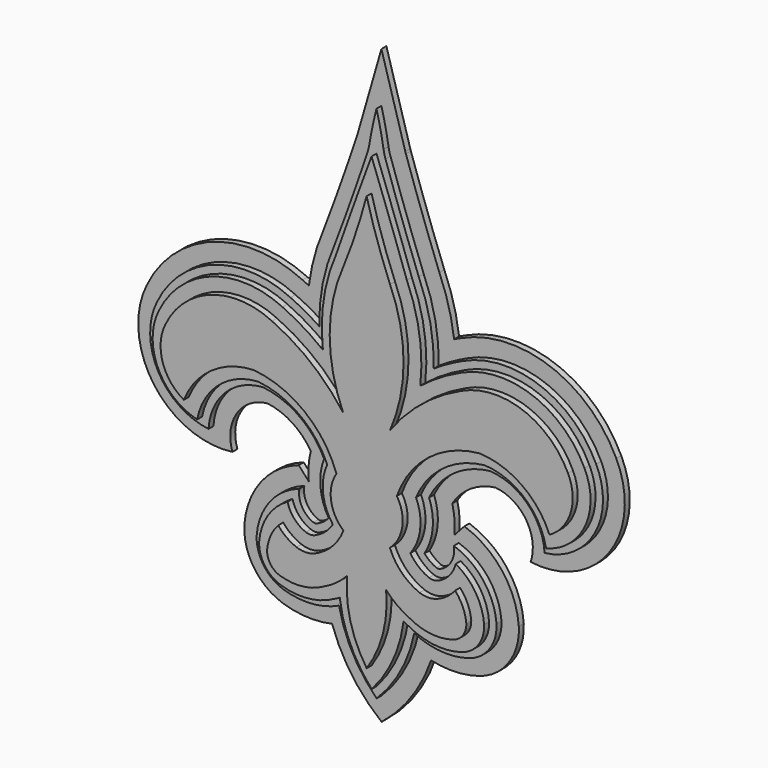
from build123d import *

# Parameters (mm, degrees)
F1_DEPTH    = 25.4
F2_DEPTH    = 19.05
F3_DEPTH    = 12.7
F4_DEPTH    = 6.35
F5_R        = 50.8
F6_T1_DEPTH = 6.35


# Not quite as in the source:
# - a fillet or chamfer that OpenCascade refuses, or shapes differently, is made with other operations: its cross-section is extruded or revolved along the edge and cut away or added


with BuildPart() as f1:
    # F0 (on Front) → F1 (new body)
    with BuildSketch(Plane.XZ):
        with BuildLine():
            ThreePointArc((-107.6217740774, 8.690867573), (-55.6471023956, -11.8476623191), (-22.9876432568, -57.196944952))
            ThreePointArc((-22.9876432568, -57.196944952), (-28.5301171317, -83.0656311724), (-15.8199295402, -106.268197298))
            ThreePointArc((-15.8199295402, -106.268197298), (-27.8174961879, -124.6891161431), (-46.1557023227, -136.8127316236))
            ThreePointArc((-46.1557023227, -136.8127316236), (-55.0099629909, -138.3229508994), (-63.864223659, -136.8127316236))
            ThreePointArc((-63.864223659, -136.8127316236), (-74.1425982594, -131.2503429818), (-82.5992301113, -123.1837123623))
            ThreePointArc((-82.5992301113, -123.1837123623), (-90.4911472712, -135.2405064996), (-94.0484032041, -149.2045521727))
            ThreePointArc((-94.0484032041, -149.2045521727), (-90.7020512597, -160.6634696416), (-81.1531394727, -167.8274869909))
            ThreePointArc((-81.1531394727, -167.8274869909), (-58.036080583, -170.2020518531), (-35.9072424478, -163.1061732759))
            ThreePointArc((-35.9072424478, -163.1061732759), (-23.0493888803, -155.5361787921), (-11.9526460775, -145.5616354935))
            ThreePointArc((-11.9526460775, -145.5616354935), (-8.6762501422, -185.8257002735), (8.0091749091, -222.6160016284))
            ThreePointArc((8.0091749091, -222.6160016284), (24.6729779001, -185.8159017262), (27.9257127936, -145.5499185811))
            ThreePointArc((27.9257127936, -145.5499185811), (39.028315047, -155.51793935), (51.8906147699, -163.0803768332))
            ThreePointArc((51.8906147699, -163.0803768332), (74.0236188538, -170.163250559), (97.1392783805, -167.77510177))
            ThreePointArc((97.1392783805, -167.77510177), (106.6839787089, -160.605474406), (110.0235964424, -149.1445924901))
            ThreePointArc((110.0235964424, -149.1445924901), (106.4581353955, -135.1826395875), (98.5591346332, -123.1304850794))
            ThreePointArc((98.5591346332, -123.1304850794), (90.1072444563, -131.2020836985), (79.8321402713, -136.7705112878))
            ThreePointArc((79.8321402713, -136.7705112878), (70.9787685859, -138.2859333548), (62.1236219925, -136.7809173918))
            ThreePointArc((62.1236219925, -136.7809173918), (43.7782947925, -124.6680801317), (31.7699054842, -106.2542146282))
            ThreePointArc((31.7699054842, -106.2542146282), (44.4664562975, -83.0441835883), (38.9087820968, -57.1787587725))
            ThreePointArc((38.9087820968, -57.1787587725), (71.541586881, -11.8102922073), (123.5041804799, 8.7587761489))
            ThreePointArc((123.5041804799, 8.7587761489), (166.7993623153, -5.6625752644), (195.2107705111, -41.3730783563))
            ThreePointArc((195.2107705111, -41.3730783563), (216.9732861452, -14.2511624984), (214.1399674952, 20.4068482921))
            ThreePointArc((214.1399674952, 20.406848292), (167.4978613851, 62.4099195769), (104.8241776257, 58.9815929048))
            ThreePointArc((104.8241776257, 58.9815929048), (64.5980000023, 34.2064244966), (31.9967480605, 0.0141343178))
            ThreePointArc((31.9967480605, 0.0141343178), (45.7550134481, 65.6656974668), (31.9195995813, 131.3010456682))
            ThreePointArc((31.9195995813, 131.3010456682), (18.7586509593, 166.8011753165), (7.884102283, 203.0670541114))
            ThreePointArc((7.884102283, 203.0670541115), (-2.9691335039, 166.7947913391), (-16.109218821, 131.2869340179))
            ThreePointArc((-16.109218821, 131.2869340178), (-29.9060608303, 65.6434670089), (-16.109218821, 0))
            ThreePointArc((-16.109218821, 0), (-48.7305576375, 34.1731267177), (-88.9712870116, 58.9246526358))
            ThreePointArc((-88.9712870116, 58.9246526358), (-151.6469745465, 62.3161496178), (-198.2643902305, 20.285677164))
            ThreePointArc((-198.2643902306, 20.285677164), (-201.0773422152, -14.3739925929), (-179.2988926172, -41.4831154048))
            ThreePointArc((-179.2988926172, -41.4831154048), (-150.9084739818, -5.7559230095), (-107.6217740774, 8.690867573))
        make_face()
    extrude(amount=F1_DEPTH)


with BuildPart() as f2:
    # F0 (on Front) → F2 (new body)
    with BuildSketch(Plane.XZ):
        with BuildLine():
            ThreePointArc((-29.8756994534, -174.8675902704), (-27.2540366228, -173.5851626194), (-24.6763913381, -172.2164108292))
            ThreePointArc((-24.6763913381, -172.2164108292), (-13.8552320974, -210.6071310198), (8.0154470243, -243.9630642074))
            ThreePointArc((8.0154470244, -243.9630642076), (29.8665213371, -210.5942848556), (40.6651190717, -172.1972124277))
            ThreePointArc((40.6651190717, -172.1972124277), (43.2435682345, -173.5644492733), (45.8659842087, -174.8453361284))
            ThreePointArc((45.8659842087, -174.8453361284), (72.9824435341, -183.3333720605), (101.2373155697, -180.3314848901))
            ThreePointArc((101.2373155697, -180.3314848901), (117.6139086806, -168.0214032355), (123.207807962, -148.3125422056))
            ThreePointArc((123.207807962, -148.3125422056), (114.3375630575, -122.0268333634), (94.1184470923, -103.0319107896))
            ThreePointArc((94.1184470923, -103.0319107896), (87.3104303405, -115.9909745964), (75.3015691391, -124.3619768951))
            ThreePointArc((75.3015691391, -124.3619768951), (71.0179091203, -125.077827485), (66.7285761619, -124.3967929812))
            ThreePointArc((66.7285761619, -124.3967929812), (55.960270597, -117.9342540793), (47.6625489032, -108.5072381948))
            ThreePointArc((47.6625489032, -108.5072381948), (57.7611970568, -83.1911033438), (53.4239364189, -56.2824142549))
            ThreePointArc((53.4239364189, -56.2824142549), (81.5889270302, -20.7682056521), (123.8857690009, -4.4739469049))
            ThreePointArc((123.8857690009, -4.4739469049), (164.7280810138, -20.7728810464), (186.6525395472, -58.8920077772))
            ThreePointArc((186.6525395472, -58.8920077772), (226.6750123427, -25.770970788), (226.0223289435, 26.1749185998))
            ThreePointArc((226.0223289435, 26.1749185998), (171.9221419751, 74.8549107017), (99.249087183, 70.9563252865))
            ThreePointArc((99.249087183, 70.9563252865), (77.767380419, 59.6132449174), (57.8415310441, 45.7175720496))
            ThreePointArc((57.8415310441, 45.7175720496), (56.970930759, 91.9956374625), (44.0833550857, 136.4515445669))
            ThreePointArc((44.0833550857, 136.4515445669), (26.2240315586, 186.4788338094), (7.8743295738, 236.3283427626))
            ThreePointArc((7.8743295738, 236.3283427626), (-10.4460760474, 186.4680595336), (-28.2759988262, 136.4302842083))
            ThreePointArc((-28.275998826, 136.4302842085), (-41.1374485351, 91.9668116204), (-41.9808541711, 45.6882426046))
            ThreePointArc((-41.9808541711, 45.6882426046), (-61.9148656556, 59.572203995), (-83.4032342743, 70.902659055))
            ThreePointArc((-83.4032342743, 70.902659055), (-156.0785674547, 74.7585387426), (-210.1501391332, 26.0467640134))
            ThreePointArc((-210.1501391332, 26.0467640134), (-210.772297323, -25.8994999436), (-170.7303684373, -58.9970127055))
            ThreePointArc((-170.7303684373, -58.9970127055), (-148.8283137299, -20.8650090302), (-107.9955865534, -4.5420774297))
            ThreePointArc((-107.9955865534, -4.5420774297), (-65.6891768482, -20.8114783615), (-37.5033217938, -56.3091301665))
            ThreePointArc((-37.5033217938, -56.3091301665), (-41.8247692607, -83.2203633251), (-31.7112462651, -108.5305595104))
            ThreePointArc((-31.7112462651, -108.5305595104), (-40.0034269046, -117.962449779), (-50.7679330119, -124.4313153721))
            ThreePointArc((-50.7679330119, -124.4313153721), (-55.0568650317, -125.1148703102), (-59.340944968, -124.401537062))
            ThreePointArc((-59.340944968, -124.401537062), (-71.3547231697, -116.0375930066), (-78.170353914, -103.0825320497))
            ThreePointArc((-78.170353914, -103.0825320497), (-98.378304353, -122.0893327552), (-107.2331013872, -148.3802495038))
            ThreePointArc((-107.2331013872, -148.3802495038), (-101.6276215028, -168.0858199734), (-85.2437974144, -180.386276083))
            ThreePointArc((-85.2437974144, -180.386276083), (-56.9871662505, -183.3715592519), (-29.8756994534, -174.8675902704))
        make_face()
        with BuildLine():
            ThreePointArc((-15.8199295402, -106.268197298), (-28.5301171317, -83.0656311724), (-22.9876432568, -57.196944952))
            ThreePointArc((-22.9876432568, -57.196944952), (-55.6471023956, -11.8476623191), (-107.6217740774, 8.690867573))
            ThreePointArc((-107.6217740774, 8.690867573), (-150.9084739818, -5.7559230095), (-179.2988926172, -41.4831154048))
            ThreePointArc((-179.2988926172, -41.4831154048), (-201.0773422152, -14.3739925929), (-198.2643902306, 20.285677164))
            ThreePointArc((-198.2643902305, 20.285677164), (-151.6469745465, 62.3161496178), (-88.9712870116, 58.9246526358))
            ThreePointArc((-88.9712870116, 58.9246526358), (-48.7305576375, 34.1731267177), (-16.109218821, 0))
            ThreePointArc((-16.109218821, 0), (-29.9060608303, 65.6434670089), (-16.109218821, 131.2869340178))
            ThreePointArc((-16.109218821, 131.2869340179), (-2.9691335039, 166.7947913391), (7.884102283, 203.0670541115))
            ThreePointArc((7.884102283, 203.0670541114), (18.7586509593, 166.8011753165), (31.9195995813, 131.3010456682))
            ThreePointArc((31.9195995813, 131.3010456682), (45.7550134481, 65.6656974668), (31.9967480605, 0.0141343178))
            ThreePointArc((31.9967480605, 0.0141343178), (64.5980000023, 34.2064244966), (104.8241776257, 58.9815929048))
            ThreePointArc((104.8241776257, 58.9815929048), (167.4978613851, 62.4099195769), (214.1399674952, 20.406848292))
            ThreePointArc((214.1399674952, 20.4068482921), (216.9732861452, -14.2511624984), (195.2107705111, -41.3730783563))
            ThreePointArc((195.2107705111, -41.3730783563), (166.7993623153, -5.6625752644), (123.5041804799, 8.7587761489))
            ThreePointArc((123.5041804799, 8.7587761489), (71.541586881, -11.8102922073), (38.9087820968, -57.1787587725))
            ThreePointArc((38.9087820968, -57.1787587725), (44.4664562975, -83.0441835883), (31.7699054842, -106.2542146282))
            ThreePointArc((31.7699054842, -106.2542146282), (43.7782947925, -124.6680801317), (62.1236219925, -136.7809173918))
            ThreePointArc((62.1236219925, -136.7809173918), (70.9787685859, -138.2859333548), (79.8321402713, -136.7705112878))
            ThreePointArc((79.8321402713, -136.7705112878), (90.1072444563, -131.2020836985), (98.5591346332, -123.1304850794))
            ThreePointArc((98.5591346332, -123.1304850794), (106.4581353955, -135.1826395875), (110.0235964424, -149.1445924901))
            ThreePointArc((110.0235964424, -149.1445924901), (106.6839787089, -160.605474406), (97.1392783805, -167.77510177))
            ThreePointArc((97.1392783805, -167.77510177), (74.0236188538, -170.163250559), (51.8906147699, -163.0803768332))
            ThreePointArc((51.8906147699, -163.0803768332), (39.028315047, -155.51793935), (27.9257127936, -145.5499185811))
            ThreePointArc((27.9257127936, -145.5499185811), (24.6729779001, -185.8159017262), (8.0091749091, -222.6160016284))
            ThreePointArc((8.0091749091, -222.6160016284), (-8.6762501422, -185.8257002735), (-11.9526460775, -145.5616354935))
            ThreePointArc((-11.9526460775, -145.5616354935), (-23.0493888803, -155.5361787921), (-35.9072424478, -163.1061732759))
            ThreePointArc((-35.9072424478, -163.1061732759), (-58.036080583, -170.2020518531), (-81.1531394727, -167.8274869909))
            ThreePointArc((-81.1531394727, -167.8274869909), (-90.7020512597, -160.6634696416), (-94.0484032041, -149.2045521727))
            ThreePointArc((-94.0484032041, -149.2045521727), (-90.4911472712, -135.2405064996), (-82.5992301113, -123.1837123623))
            ThreePointArc((-82.5992301113, -123.1837123623), (-74.1425982594, -131.2503429818), (-63.864223659, -136.8127316236))
            ThreePointArc((-63.864223659, -136.8127316236), (-55.0099629909, -138.3229508994), (-46.1557023227, -136.8127316236))
            ThreePointArc((-46.1557023227, -136.8127316236), (-27.8174961879, -124.6891161431), (-15.8199295402, -106.268197298))
        make_face(mode=Mode.SUBTRACT)
    extrude(amount=F2_DEPTH)


with BuildPart() as f3:
    # F0 (on Front) → F3 (new body)
    with BuildSketch(Plane.XZ):
        with BuildLine():
            ThreePointArc((-87.600157757, -187.6328630649), (-58.6890196944, -191.1595322399), (-30.5161688034, -183.7715844727))
            ThreePointArc((-30.5161688034, -183.7715844727), (-16.5641396659, -222.2571523724), (8.0186871126, -254.9906624378))
            ThreePointArc((8.0186871126, -254.9906624378), (32.5822743698, -222.2427123542), (46.5116857251, -183.7489524324))
            ThreePointArc((46.5116857251, -183.7489524324), (74.6888731507, -191.1203436391), (103.5979338359, -187.5766859465))
            ThreePointArc((103.5979338359, -187.5766859465), (123.9214936647, -172.2969470055), (130.8127999617, -147.8219106676))
            ThreePointArc((130.8127999617, -147.8219106676), (117.3819058972, -113.1531384715), (87.0814905999, -91.6078950575))
            ThreePointArc((87.0814905999, -91.6078950575), (84.4380090885, -106.945760837), (72.7202350562, -117.1893877777))
            ThreePointArc((72.7202350562, -117.1893877777), (71.0254392186, -117.4576091576), (69.325337641, -117.2253802503))
            ThreePointArc((69.325337641, -117.2253802503), (62.6513057826, -113.4881207497), (57.0078989345, -108.324617194))
            ThreePointArc((57.0078989345, -108.324617194), (65.4476371393, -82.9101925594), (61.7356254368, -56.3895754927))
            ThreePointArc((61.7356254368, -56.3895754927), (87.1596792608, -26.1437180593), (124.0968865754, -12.1138527528))
            ThreePointArc((124.0968865754, -12.1138527528), (162.717750006, -29.2997135624), (180.0993877199, -67.8328625937))
            ThreePointArc((180.0993877199, -67.8328625937), (231.6610200117, -32.8154530476), (232.8782812268, 29.5009907779))
            ThreePointArc((232.8782812268, 29.5009907779), (174.4766768488, 82.0339790462), (96.0350501352, 77.8658321143))
            ThreePointArc((96.0350501352, 77.8658321143), (80.9486418346, 70.2808614935), (66.5375562041, 61.4801736977))
            ThreePointArc((66.5375562041, 61.4801736977), (63.0978299131, 101.2017138745), (51.1773603835, 139.2481969861))
            ThreePointArc((51.1773603835, 139.2481969861), (32.9209394192, 188.665796547), (15.7474019582, 238.4700700971))
            ThreePointArc((15.7474019582, 238.4700700971), (12.307760344, 257.7334068671), (7.8624413353, 276.7898078091))
            ThreePointArc((7.8624413353, 276.7898078091), (3.4283212561, 257.7307979431), (0, 238.4654432535))
            ThreePointArc((0, 238.4654432535), (-17.1442678824, 188.6510865723), (-35.3716463032, 139.2227674761))
            ThreePointArc((-35.3716463032, 139.2227674761), (-47.2697564218, 101.1692860771), (-50.6861404479, 61.4457314633))
            ThreePointArc((-50.6861404479, 61.4457314633), (-65.1023951611, 70.2379493162), (-80.1932580327, 77.8140533625))
            ThreePointArc((-80.1932580327, 77.8140533625), (-158.6373205418, 81.9361047195), (-217.0080447412, 29.3688068361))
            ThreePointArc((-217.0080447412, 29.3688068361), (-215.7541645639, -32.9469109277), (-164.1719638039, -67.934015133))
            ThreePointArc((-164.1719638039, -67.934015133), (-146.8129724247, -29.3906587381), (-108.202214634, -12.1821060184))
            ThreePointArc((-108.202214634, -12.1821060184), (-71.2567692908, -26.1902633962), (-45.8149464054, -56.4211756053))
            ThreePointArc((-45.8149464054, -56.4211756053), (-49.5113730885, -82.9439693919), (-41.056701997, -108.3534301735))
            ThreePointArc((-41.056701997, -108.3534301735), (-46.6970736278, -113.5202490874), (-53.3689081985, -117.2614298213))
            ThreePointArc((-53.3689081985, -117.2614298213), (-55.0688730173, -117.4946577236), (-56.7638261779, -117.2274323072))
            ThreePointArc((-56.7638261779, -117.2274323072), (-68.4876176759, -106.9906928809), (-71.1401117605, -91.6543831454))
            ThreePointArc((-71.1401117605, -91.6543831454), (-101.4278611394, -113.2174283506), (-114.838380385, -147.8940869918))
            ThreePointArc((-114.838380385, -147.8940869918), (-107.9326929491, -172.3650695479), (-87.600157757, -187.6328630649))
        make_face()
        with BuildLine():
            ThreePointArc((8.0154470243, -243.9630642074), (-13.8552320974, -210.6071310198), (-24.6763913381, -172.2164108292))
            ThreePointArc((-24.6763913381, -172.2164108292), (-27.2540366228, -173.5851626194), (-29.8756994534, -174.8675902704))
            ThreePointArc((-29.8756994534, -174.8675902704), (-56.9871662505, -183.3715592519), (-85.2437974144, -180.386276083))
            ThreePointArc((-85.2437974144, -180.386276083), (-101.6276215028, -168.0858199734), (-107.2331013872, -148.3802495038))
            ThreePointArc((-107.2331013872, -148.3802495038), (-98.378304353, -122.0893327552), (-78.170353914, -103.0825320497))
            ThreePointArc((-78.170353914, -103.0825320497), (-71.3547231697, -116.0375930066), (-59.340944968, -124.401537062))
            ThreePointArc((-59.340944968, -124.401537062), (-55.0568650317, -125.1148703102), (-50.7679330119, -124.4313153721))
            ThreePointArc((-50.7679330119, -124.4313153721), (-40.0034269046, -117.962449779), (-31.7112462651, -108.5305595104))
            ThreePointArc((-31.7112462651, -108.5305595104), (-41.8247692607, -83.2203633251), (-37.5033217938, -56.3091301665))
            ThreePointArc((-37.5033217938, -56.3091301665), (-65.6891768482, -20.8114783615), (-107.9955865534, -4.5420774297))
            ThreePointArc((-107.9955865534, -4.5420774297), (-148.8283137299, -20.8650090302), (-170.7303684373, -58.9970127055))
            ThreePointArc((-170.7303684373, -58.9970127055), (-210.772297323, -25.8994999436), (-210.1501391332, 26.0467640134))
            ThreePointArc((-210.1501391332, 26.0467640134), (-156.0785674547, 74.7585387426), (-83.4032342743, 70.902659055))
            ThreePointArc((-83.4032342743, 70.902659055), (-61.9148656556, 59.572203995), (-41.9808541711, 45.6882426046))
            ThreePointArc((-41.9808541711, 45.6882426046), (-41.1374485351, 91.9668116204), (-28.275998826, 136.4302842085))
            ThreePointArc((-28.2759988262, 136.4302842083), (-10.4460760474, 186.4680595336), (7.8743295738, 236.3283427626))
            ThreePointArc((7.8743295738, 236.3283427626), (26.2240315586, 186.4788338094), (44.0833550857, 136.4515445669))
            ThreePointArc((44.0833550857, 136.4515445669), (56.970930759, 91.9956374625), (57.8415310441, 45.7175720496))
            ThreePointArc((57.8415310441, 45.7175720496), (77.767380419, 59.6132449174), (99.249087183, 70.9563252865))
            ThreePointArc((99.249087183, 70.9563252865), (171.9221419751, 74.8549107017), (226.0223289435, 26.1749185998))
            ThreePointArc((226.0223289435, 26.1749185998), (226.6750123427, -25.770970788), (186.6525395472, -58.8920077772))
            ThreePointArc((186.6525395472, -58.8920077772), (164.7280810138, -20.7728810464), (123.8857690009, -4.4739469049))
            ThreePointArc((123.8857690009, -4.4739469049), (81.5889270302, -20.7682056521), (53.4239364189, -56.2824142549))
            ThreePointArc((53.4239364189, -56.2824142549), (57.7611970568, -83.1911033438), (47.6625489032, -108.5072381948))
            ThreePointArc((47.6625489032, -108.5072381948), (55.960270597, -117.9342540793), (66.7285761619, -124.3967929812))
            ThreePointArc((66.7285761619, -124.3967929812), (71.0179091203, -125.077827485), (75.3015691391, -124.3619768951))
            ThreePointArc((75.3015691391, -124.3619768951), (87.3104303405, -115.9909745964), (94.1184470923, -103.0319107896))
            ThreePointArc((94.1184470923, -103.0319107896), (114.3375630575, -122.0268333634), (123.207807962, -148.3125422056))
            ThreePointArc((123.207807962, -148.3125422056), (117.6139086806, -168.0214032355), (101.2373155697, -180.3314848901))
            ThreePointArc((101.2373155697, -180.3314848901), (72.9824435341, -183.3333720605), (45.8659842087, -174.8453361284))
            ThreePointArc((45.8659842087, -174.8453361284), (43.2435682345, -173.5644492733), (40.6651190717, -172.1972124277))
            ThreePointArc((40.6651190717, -172.1972124277), (29.8665213371, -210.5942848556), (8.0154470244, -243.9630642076))
        make_face(mode=Mode.SUBTRACT)
    extrude(amount=F3_DEPTH)

    # F5
    f5_edges = [f3.edges().sort_by_distance(p)[0] for p in [
        (0, -6.35, 238.465443),
        (15.747402, -6.35, 238.47007),
    ]]
    fillet(f5_edges, radius=F5_R)


with BuildPart() as f4:
    # F0 (on Front) → F4 (new body)
    with BuildSketch(Plane.XZ):
        with BuildLine():
            ThreePointArc((-108.6274055535, -29.5264491572), (-83.3357301656, -38.8625080934), (-64.5055984949, -58.1564704043))
            ThreePointArc((-64.5055984949, -58.1564704043), (-66.8260443975, -72.0360587705), (-66.5492699145, -86.1055590561))
            Line((-66.5492699145, -86.1055590561), (-76.853644502, -74.8174041572))
            ThreePointArc((-76.853644502, -74.8174041572), (-115.5382303483, -102.3991039034), (-132.5825060803, -146.747046446))
            ThreePointArc((-132.5825060803, -146.747046446), (-122.6466718611, -182.3466630871), (-93.0937328561, -204.5429984333))
            ThreePointArc((-93.0937328561, -204.5429984333), (-68.0400358181, -209.0273403938), (-42.6927754052, -206.7222487136))
            ThreePointArc((-42.6927754052, -206.7222487136), (-22.5050376802, -246.3638663092), (8.0256589964, -278.7193783663))
            ThreePointArc((8.0256589964, -278.7193783663), (38.5373372489, -246.3459310636), (58.7017767825, -206.6924573401))
            ThreePointArc((58.7017767825, -206.6924573401), (84.050387366, -208.9826537464), (109.1014449329, -204.4835901915))
            ThreePointArc((109.1014449329, -204.4835901915), (138.6413355457, -182.2698924081), (148.5562485549, -146.6644432935))
            ThreePointArc((148.5562485549, -146.6644432935), (131.4859154701, -102.3265241795), (92.7851283976, -74.7675615183))
            Line((92.7851283976, -74.7675615183), (82.4873888767, -86.0617696545))
            ThreePointArc((82.4873888767, -86.0617696545), (82.7558956152, -71.9921091563), (80.4272940151, -58.1138867561))
            ThreePointArc((80.4272940151, -58.1138867561), (99.2460846738, -38.8088625777), (124.5322695226, -29.4579430411))
            ThreePointArc((124.5322695226, -29.4579430411), (156.0798030587, -48.3525346549), (160.7192167762, -84.8316835597))
            ThreePointArc((160.7192167762, -84.8316835597), (241.1081953363, -50.1915165247), (248.4196811451, 37.0373274515))
            ThreePointArc((248.4196811451, 37.0373274515), (180.2708430385, 98.3051536723), (88.754706774, 93.5294371469))
            ThreePointArc((88.754706774, 93.5294371469), (85.5183904122, 92.0314638174), (82.3065204933, 90.4817672942))
            ThreePointArc((82.3065204933, 90.4817672942), (76.7187719724, 118.6748058083), (67.170165449, 145.7837428522))
            ThreePointArc((67.170165449, 145.7837428522), (49.3650157886, 193.9758196787), (32.5970673662, 242.5385165661))
            ThreePointArc((32.5970673662, 242.5385165661), (20.2120968482, 285.3061966761), (7.8473715181, 328.0797343394))
            ThreePointArc((7.8473715182, 328.0797343393), (-4.4922165529, 285.2989381458), (-16.8520532505, 242.5239876078))
            ThreePointArc((-16.8520532505, 242.5239876078), (-33.5914617552, 193.9514457123), (-51.3682891071, 145.7489143205))
            ThreePointArc((-51.3682891071, 145.7489143205), (-60.9009638874, 118.6343708848), (-66.4721442957, 90.4380536954))
            ThreePointArc((-66.4721442957, 90.4380536954), (-69.6849243122, 91.9858625516), (-72.9221203732, 93.4819338576))
            ThreePointArc((-72.9221203732, 93.4819338576), (-164.4410472034, 98.2038716956), (-232.5538705732, 36.8960095757))
            ThreePointArc((-232.5538705732, 36.8960095757), (-225.1911275165, -50.3285228726), (-144.7818071454, -84.9214447443))
            ThreePointArc((-144.7818071454, -84.9214447443), (-140.1638305651, -48.4395758672), (-108.6274055535, -29.5264491572))
        make_face()
        with BuildLine():
            ThreePointArc((8.0186871126, -254.9906624378), (-16.5641396659, -222.2571523724), (-30.5161688034, -183.7715844727))
            ThreePointArc((-30.5161688034, -183.7715844727), (-58.6890196944, -191.1595322399), (-87.600157757, -187.6328630649))
            ThreePointArc((-87.600157757, -187.6328630649), (-107.9326929491, -172.3650695479), (-114.838380385, -147.8940869918))
            ThreePointArc((-114.838380385, -147.8940869918), (-101.4278611394, -113.2174283506), (-71.1401117605, -91.6543831454))
            ThreePointArc((-71.1401117605, -91.6543831454), (-68.4876176759, -106.9906928809), (-56.7638261779, -117.2274323072))
            ThreePointArc((-56.7638261779, -117.2274323072), (-55.0688730173, -117.4946577236), (-53.3689081985, -117.2614298213))
            ThreePointArc((-53.3689081985, -117.2614298213), (-46.6970736278, -113.5202490874), (-41.056701997, -108.3534301735))
            ThreePointArc((-41.056701997, -108.3534301735), (-49.5113730885, -82.9439693919), (-45.8149464054, -56.4211756053))
            ThreePointArc((-45.8149464054, -56.4211756053), (-71.2567692908, -26.1902633962), (-108.202214634, -12.1821060184))
            ThreePointArc((-108.202214634, -12.1821060184), (-146.8129724247, -29.3906587381), (-164.1719638039, -67.934015133))
            ThreePointArc((-164.1719638039, -67.934015133), (-215.7541645639, -32.9469109277), (-217.0080447412, 29.3688068361))
            ThreePointArc((-217.0080447412, 29.3688068361), (-158.6373205418, 81.9361047195), (-80.1932580327, 77.8140533625))
            ThreePointArc((-80.1932580327, 77.8140533625), (-65.1023951611, 70.2379493162), (-50.6861404479, 61.4457314633))
            ThreePointArc((-50.6861404479, 61.4457314633), (-47.2697564218, 101.1692860771), (-35.3716463032, 139.2227674761))
            ThreePointArc((-35.3716463032, 139.2227674761), (-17.1442678824, 188.6510865723), (0, 238.4654432535))
            ThreePointArc((0, 238.4654432535), (3.4283212561, 257.7307979431), (7.8624413353, 276.7898078091))
            ThreePointArc((7.8624413353, 276.7898078091), (12.307760344, 257.7334068671), (15.7474019582, 238.4700700971))
            ThreePointArc((15.7474019582, 238.4700700971), (32.9209394192, 188.665796547), (51.1773603835, 139.2481969861))
            ThreePointArc((51.1773603835, 139.2481969861), (63.0978299131, 101.2017138745), (66.5375562041, 61.4801736977))
            ThreePointArc((66.5375562041, 61.4801736977), (80.9486418346, 70.2808614935), (96.0350501352, 77.8658321143))
            ThreePointArc((96.0350501352, 77.8658321143), (174.4766768488, 82.0339790462), (232.8782812268, 29.5009907779))
            ThreePointArc((232.8782812268, 29.5009907779), (231.6610200117, -32.8154530476), (180.0993877199, -67.8328625937))
            ThreePointArc((180.0993877199, -67.8328625937), (162.717750006, -29.2997135624), (124.0968865754, -12.1138527528))
            ThreePointArc((124.0968865754, -12.1138527528), (87.1596792608, -26.1437180593), (61.7356254368, -56.3895754927))
            ThreePointArc((61.7356254368, -56.3895754927), (65.4476371393, -82.9101925594), (57.0078989345, -108.324617194))
            ThreePointArc((57.0078989345, -108.324617194), (62.6513057826, -113.4881207497), (69.325337641, -117.2253802503))
            ThreePointArc((69.325337641, -117.2253802503), (71.0254392186, -117.4576091576), (72.7202350562, -117.1893877777))
            ThreePointArc((72.7202350562, -117.1893877777), (84.4380090885, -106.945760837), (87.0814905999, -91.6078950575))
            ThreePointArc((87.0814905999, -91.6078950575), (117.3819058972, -113.1531384715), (130.8127999617, -147.8219106676))
            ThreePointArc((130.8127999617, -147.8219106676), (123.9214936647, -172.2969470055), (103.5979338359, -187.5766859465))
            ThreePointArc((103.5979338359, -187.5766859465), (74.6888731507, -191.1203436391), (46.5116857251, -183.7489524324))
            ThreePointArc((46.5116857251, -183.7489524324), (32.5822743698, -222.2427123542), (8.0186871126, -254.9906624378))
        make_face(mode=Mode.SUBTRACT)
    extrude(amount=F4_DEPTH)

    # F6: fillet of radius 50.8 on 2 edges, made by hand

    # F6_s2 → F6_t1 (join)
    with BuildSketch(Plane.XZ):
        with BuildLine():
            ThreePointArc((-16.5707171409, 243.4967924994), (-16.8632638471, 242.5219069038), (-17.1752837548, 241.5530781898))
            ThreePointArc((-17.1752837548, 241.5530781898), (-17.0136166792, 242.0385156459), (-16.8520532505, 242.5239876078))
            ThreePointArc((-16.8520532505, 242.5239876078), (-16.7113838865, 243.010389675), (-16.5707171409, 243.4967924994))
        make_face()
        with BuildLine():
            ThreePointArc((32.920868353, 241.5677972555), (32.6082791839, 242.5364424492), (32.3151596536, 243.5111559665))
            ThreePointArc((32.3151596536, 243.5111559665), (32.456112201, 243.0248358869), (32.5970673662, 242.5385165661))
            ThreePointArc((32.5970673662, 242.5385165661), (32.7589160463, 242.0531396275), (32.920868353, 241.5677972555))
        make_face()
    extrude(amount=F6_T1_DEPTH)


solid = Compound([f1.part, f2.part, f3.part, f4.part])
